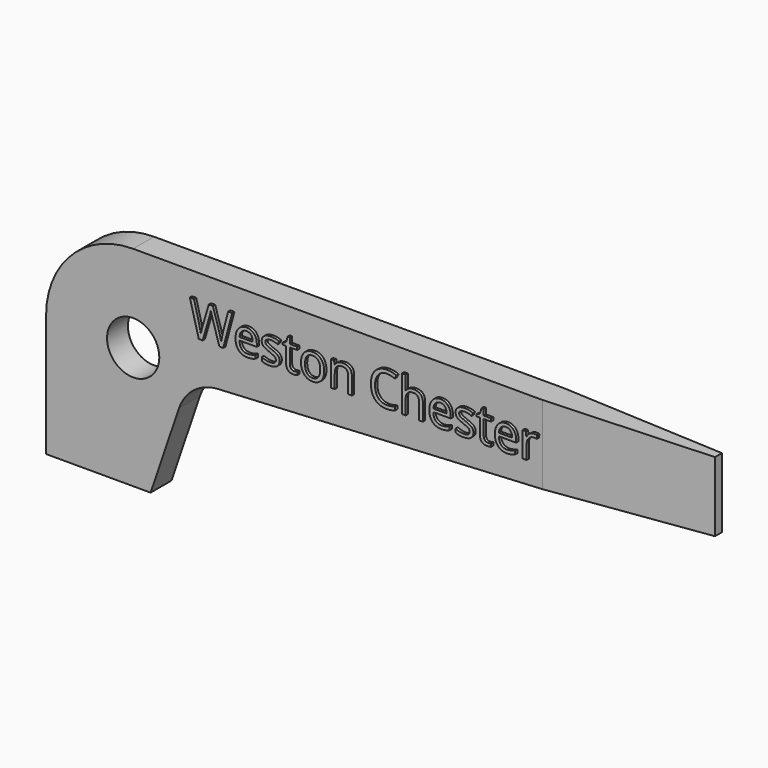
from build123d import *

# Parameters (mm, degrees)
F1_DEPTH     = 2.38125
F2_R         = 2.38125
F3_DEPTH     = 2.38225
F5_DEPTH     = 19.051
F6_TEXT_SIZE = 4.294447837
F7_DEPTH     = 0.254


# Not quite as in the source:
# - Text() gives the source's letters only with a copy of the font that has no kerning and outlines rounded to 1/6400 em; it was checked with that copy


with BuildPart() as f1:
    # F0 (on Front) → F1 (new body)
    with BuildSketch(Plane.XZ):
        with BuildLine():
            Line((60.325, 19.05), (7.9375, 19.05))
            ThreePointArc((7.9375, 19.05), (2.3248399243, 16.7251600757), (0, 11.1125))
            Line((0, 11.1125), (0, 0))
            Line((0, 0), (9.525, 0))
            Line((9.525, 0), (12.1173647876, 7.6271664624))
            ThreePointArc((12.1173647876, 7.6271664624), (13.4786145605, 9.5135918491), (15.6631963617, 10.3130942181))
            Line((15.6631963617, 10.3130942181), (60.325, 12.7))
            Line((60.325, 12.7), (60.325, 19.05))
        make_face()
    extrude(amount=F1_DEPTH)

    # F2 (on face) → F3 (cut, through all)
    with BuildSketch(Plane.XZ.offset(2.38125)):
        with Locations((7.9375, 11.1125)):
            Circle(F2_R)
    extrude(amount=-F3_DEPTH, mode=Mode.SUBTRACT)

    # F4 (on face) → F5 (cut, through all)
    with BuildSketch(Plane.XY.offset(19.05)):
        Polygon((60.325, 0), (45.24375, 0), (60.325, -0.79375), align=None)
        Polygon((60.325, -2.38125), (60.325, -1.5875), (45.24375, -2.38125), align=None)
    extrude(amount=-F5_DEPTH, mode=Mode.SUBTRACT)

    # F6 (on face) → F7 (join)
    with BuildSketch(Plane.XZ.offset(2.38125)):
        with Locations((13.2487715997, 13.9259975574)):
            Text('Weston Chester', F6_TEXT_SIZE, font='Open Sans', text_align=(TextAlign.LEFT, TextAlign.BOTTOM))
    extrude(amount=F7_DEPTH)


solid = f1.part
